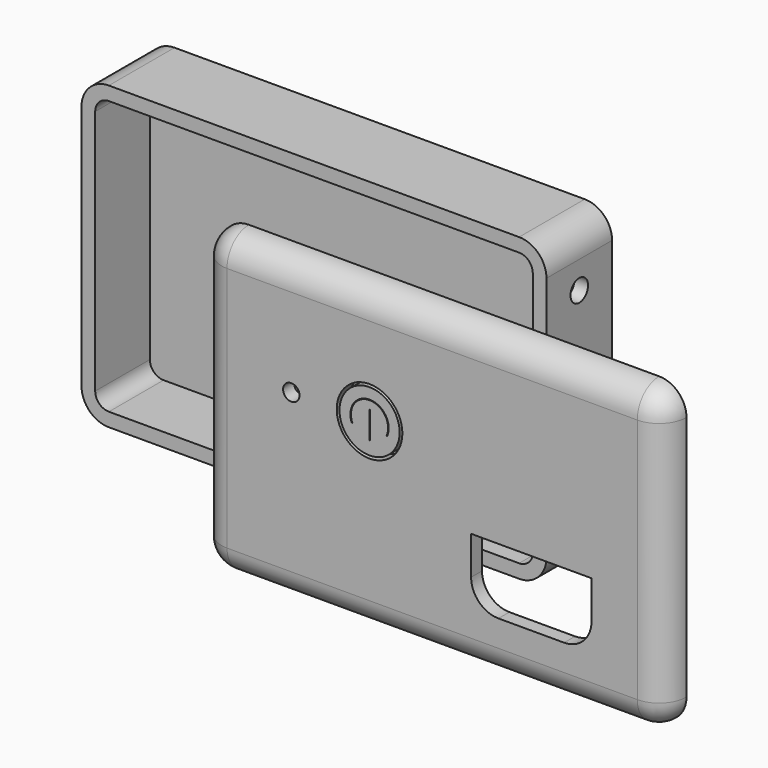
from build123d import *

# Parameters (mm, degrees)
F0_W      = 85
F0_H      = 55
F1_DEPTH  = 7.5
F2_R      = 5
F3_T      = -2.5
F4_W      = 5
F4_H      = 10
F5_DEPTH  = 25
F6_R      = 2
F7_DEPTH  = 25
F9_DEPTH  = 85
F10_T     = -2.5
F11_R     = 6
F11_R_2   = 5.5
F11_R_3   = 1.5
F12_DEPTH = 25
F14_DEPTH = 25
F15_W     = 0.1
F15_H     = 5
F16_DEPTH = 25
F17_R     = 4.99999


# Not quite as in the source:
# - a fillet or chamfer is up to 0.001 mm smaller than in the source, because OpenCascade refuses the exact size


with BuildPart() as f1:
    # F0 (on Front) → F1 (new body, symmetric)
    with BuildSketch(Plane.XZ):
        Rectangle(F0_W, F0_H)
    extrude(amount=F1_DEPTH, both=True)

    # F2
    f2_edges = [f1.edges().sort_by_distance(p)[0] for p in [
        (-42.5, 0, 27.5),
        (42.5, 0, 27.5),
        (42.5, 0, -27.5),
        (-42.5, 0, -27.5),
    ]]
    fillet(f2_edges, radius=F2_R)

    # F3
    f3_openings = [f1.faces().sort_by_distance(p)[0] for p in [
        (0, -7.5, 0),
    ]]
    offset(amount=F3_T, openings=f3_openings)

    # F4 (on face) → F5 (cut)
    with BuildSketch(Plane.YZ.offset(42.5)):
        with Locations((0, -15.5)):
            Rectangle(F4_W, F4_H)
        with Locations((0, -0.5)):
            Rectangle(F4_W, F4_H)
    extrude(amount=-F5_DEPTH, mode=Mode.SUBTRACT)

    # F6 (on face) → F7 (cut)
    with BuildSketch(Plane.YZ.offset(42.5)):
        with Locations((0, 17.5)):
            Circle(F6_R)
    extrude(amount=-F7_DEPTH, mode=Mode.SUBTRACT)


with BuildPart() as f9:
    # F8 (on Right) → F9 (new body)
    with BuildSketch(Plane.YZ):
        with BuildLine():
            Line((-28.6249992251, -27.5), (-28.6249992251, 27.5))
            ThreePointArc((-28.6249992251, 27.5), (-32.1605331311, 26.0355339059), (-33.6249992251, 22.5))
            Line((-33.6249992251, 22.5), (-33.6249992251, -22.5))
            ThreePointArc((-33.6249992251, -22.5), (-32.1605331311, -26.0355339059), (-28.6249992251, -27.5))
        make_face()
    extrude(amount=F9_DEPTH)

    # F10
    f10_openings = [f9.faces().sort_by_distance(p)[0] for p in [
        (42.5, -28.624999, 0),
    ]]
    offset(amount=F10_T, openings=f10_openings)

    # F11 (on face) → F12 (cut)
    with BuildSketch(Plane.XZ.offset(33.6249992251)):
        with Locations((31.0585959434, 6.3749989495)):
            Circle(F11_R)
        with Locations((31.0585959434, 6.3749989495)):
            Circle(F11_R_2, mode=Mode.SUBTRACT)
        with Locations((16.7558868038, 6.3749989495)):
            Circle(F11_R_3)
    extrude(amount=-F12_DEPTH, mode=Mode.SUBTRACT)

    # F13 (on face) → F14 (cut)
    with BuildSketch(Plane.XZ.offset(33.6249992251)):
        with BuildLine():
            Line((71.6250017881, -5.6888253678), (49.6250017881, -5.6888253678))
            Line((49.6250017881, -5.6888253678), (49.6250017881, -12.6888253678))
            ThreePointArc((49.6250017881, -12.6888253678), (51.0894678822, -16.2243592737), (54.6250017881, -17.6888253678))
            Line((54.6250017881, -17.6888253678), (66.6250017881, -17.6888253678))
            ThreePointArc((66.6250017881, -17.6888253678), (70.1605356941, -16.2243592737), (71.6250017881, -12.6888253678))
            Line((71.6250017881, -12.6888253678), (71.6250017881, -5.6888253678))
        make_face()
    extrude(amount=-F14_DEPTH, mode=Mode.SUBTRACT)

    # F15 (on face) → F16 (cut)
    with BuildSketch(Plane.XZ.offset(33.6249992251)):
        with BuildLine():
            Line((34.1992405995, 5.0725584924), (34.261399235, 4.9635985542))
            ThreePointArc((34.261399235, 4.9635985542), (31.0585959434, 9.8749989495), (27.8557926519, 4.9635985542))
            Line((27.8557926519, 4.9635985542), (27.9179512873, 5.0725584924))
            ThreePointArc((27.9179512873, 5.0725584924), (31.0585959434, 9.7749989495), (34.1992405995, 5.0725584924))
        make_face()
        with Locations((31.0585959434, 5.8176338766)):
            Rectangle(F15_W, F15_H)
    extrude(amount=-F16_DEPTH, mode=Mode.SUBTRACT)

    # F17 (radius 5 in the source; OpenCascade refuses exactly that, so slightly less here)
    f17_edges = [f9.edges().sort_by_distance(p)[0] for p in [
        (0, -32.160533, 26.035534),
        (85, -33.624999, 0),
    ]]
    fillet(f17_edges, radius=F17_R)


solid = Compound([f1.part, f9.part])
